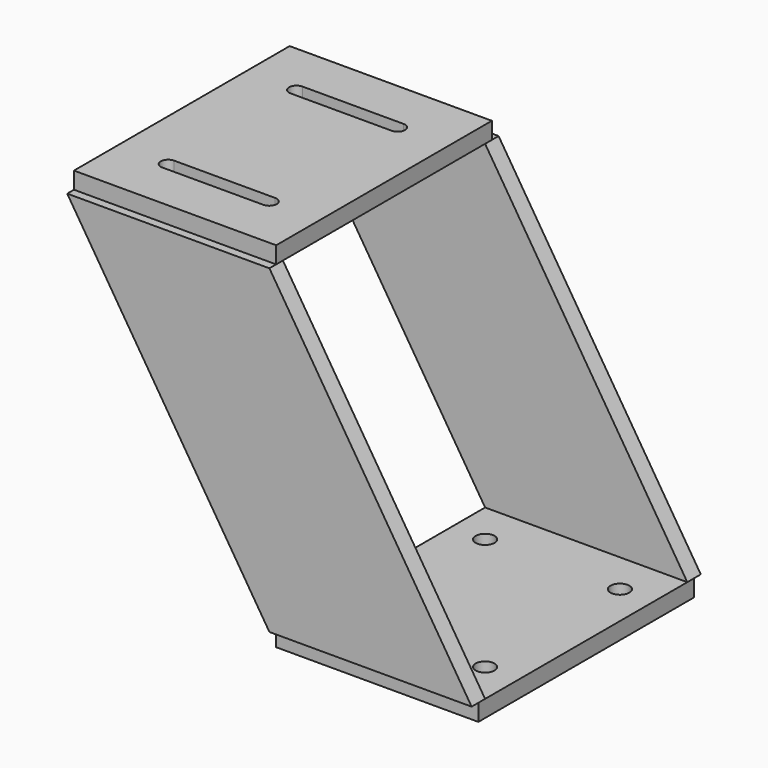
from build123d import *

# Parameters (mm, degrees)
F0_W      = 152.4
F0_H      = 203.2
F1_DEPTH  = 12.7
F3_D      = 14.2875
F5_W      = 152.4
F5_H      = 203.2
F6_DEPTH  = 12.7
F8_DEPTH  = 266.701
F10_DEPTH = 6.35


# Not quite as in the source:
# - a length typed as a fraction of an inch, garbled in the dataset ("3 / 203.2 mm" for 3/8 in), is restored


with BuildPart() as f1:
    # F0 (on Top) → F1 (new body)
    with BuildSketch(Plane.XY):
        Rectangle(F0_W, F0_H)
    extrude(amount=F1_DEPTH)

    # F3 (through all)
    with Locations(Plane.XY.offset(12.7)):
        with Locations((-50.8, 63.5), (50.8, 63.5), (-50.8, -63.5), (50.8, -63.5)):
            Hole(F3_D / 2)


with BuildPart() as f6:
    # F5 (on offset) → F6 (new body)
    with BuildSketch(Plane(origin=(0, 0, 266.7), x_dir=(1, 0, 0), z_dir=(0, 0, -1))):
        with Locations((-152.4, 0)):
            Rectangle(F5_W, F5_H)
    extrude(amount=F6_DEPTH)

    # F7 (on face) → F8 (cut, through all)
    with BuildSketch(Plane.XY.offset(266.7)):
        with BuildLine():
            ThreePointArc((-190.5, -54.864), (-196.088, -60.452), (-190.5, -66.04))
            Line((-190.5, -66.04), (-114.3, -66.04))
            ThreePointArc((-114.3, -66.04), (-108.712, -60.452), (-114.3, -54.864))
            Line((-114.3, -54.864), (-190.5, -54.864))
        make_face()
        with BuildLine():
            Line((-190.5, 54.864), (-114.3, 54.864))
            ThreePointArc((-114.3, 54.864), (-108.712, 60.452), (-114.3, 66.04))
            Line((-114.3, 66.04), (-190.5, 66.04))
            ThreePointArc((-190.5, 66.04), (-196.088, 60.452), (-190.5, 54.864))
        make_face()
    extrude(amount=-F8_DEPTH, mode=Mode.SUBTRACT)


with BuildPart() as f10:
    # F9 (on face) → F10 (new body, symmetric)
    with BuildSketch(Plane.XZ.offset(101.6)):
        Polygon((-76.2, 254), (-228.6, 254), (-76.2, 12.7), (76.2, 12.7), align=None)
    extrude(amount=F10_DEPTH, both=True)


with BuildPart() as f11_1:
    # F11: instance of F10
    add(f10.part.mirror(Plane.XZ))


solid = Compound([f1.part, f6.part, f10.part, f11_1.part])
